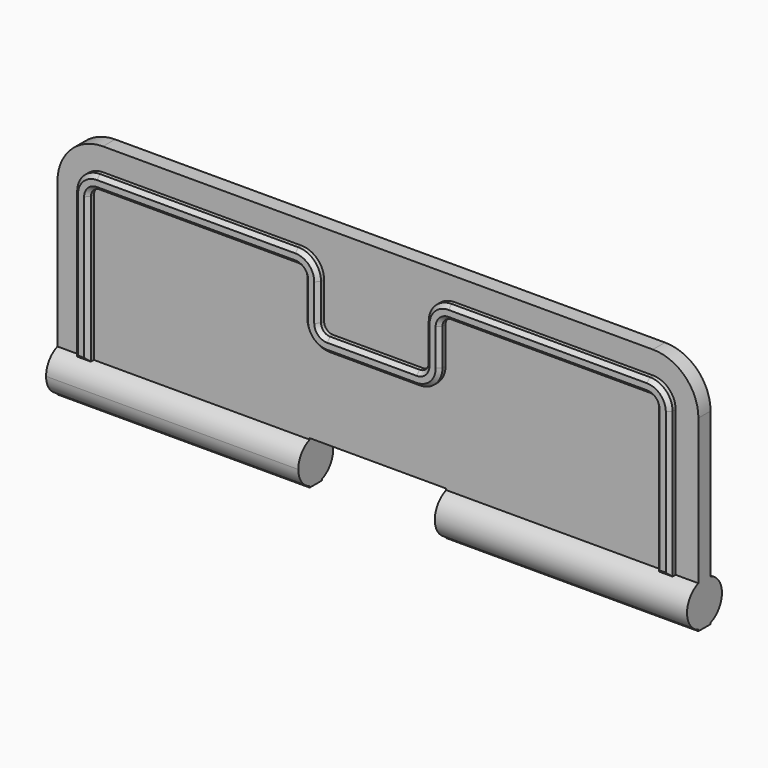
from build123d import *

# Parameters (mm, degrees)
F0_W     = 33.259
F0_H     = 5.75
F1_DEPTH = 2
F3_DEPTH = 33.259
F6_DEPTH = 33.259
F4_W     = 1.8128321722
F4_H     = 19.1795176684
F4_W_2   = 26.160747505
F4_H_2   = 1.8128321722
F4_H_3   = 4.8250346239
F4_W_3   = 5.911082495
F4_H_4   = 1.81283
F7_DEPTH = 1
F8_SIZE  = 0.5


# Not quite as in the source:
# - ends of sketch curves that miss each other by under 0.0002 mm in the source are joined
# - a pattern or mirror of a feature is missing from the dataset's text; its kind, count and spacing are read off the source's solid


with BuildPart() as f1:
    # F0 (on Front) → F1 (new body)
    with BuildSketch(Plane.XZ):
        with BuildLine():
            Line((36.259, 12.5), (-36.259, 12.5))
            ThreePointArc((-36.259, 12.5), (-40.5016406871, 10.7426406871), (-42.259, 6.5))
            Line((-42.259, 6.5), (-42.259, -12.5))
            Line((-42.259, -12.5), (-9, -12.5))
            Line((-9, -12.5), (-3.6677482234, -11.0712274426))
            Line((-3.6677482234, -11.0712274426), (3.6677482234, -11.0712274426))
            Line((3.6677482234, -11.0712274426), (9, -12.5))
            Line((9, -12.5), (42.259, -12.5))
            Line((42.259, -12.5), (42.259, 6.5))
            ThreePointArc((42.259, 6.5), (40.5016406871, 10.7426406871), (36.259, 12.5))
        make_face()
        with Locations((-25.6295, -15.375)):
            Rectangle(F0_W, F0_H)
        with Locations((25.6295, -15.375)):
            Rectangle(F0_W, F0_H)
        Polygon((-3.6677482234, -11.0712274426), (-9, -12.5), (9, -12.5), (3.6677482234, -11.0712274426), align=None)
    extrude(amount=F1_DEPTH)

    # F2 (on face) → F3 (join, through all)
    with BuildSketch(Plane(origin=(-42.259, 0, 0), x_dir=(0, -1, 0), z_dir=(-1, 0, 0))):
        with BuildLine():
            ThreePointArc((3.875, -15.375), (3.3601509486, -13.7332593079), (2, -12.6795176684))
            Line((2, -12.6795176684), (2, -18.0704823316))
            ThreePointArc((2, -18.0704823316), (3.3601509486, -17.0167406921), (3.875, -15.375))
        make_face()
        with BuildLine():
            Line((2, -18.0704823316), (2, -12.6795176684))
            ThreePointArc((2, -12.6795176684), (-1.875, -15.375), (2, -18.0704823316))
        make_face()
    extrude(amount=-F3_DEPTH)

    # F5 (on face) → F6 (join, through all)
    with BuildSketch(Plane.YZ.offset(42.259)):
        with BuildLine():
            ThreePointArc((0, -18.0704823316), (1.875, -15.375), (0, -12.6795176684))
            Line((0, -12.6795176684), (0, -12.5))
            Line((0, -12.5), (-2, -12.5))
            Line((-2, -12.5), (-2, -12.6795176684))
            ThreePointArc((-2, -12.6795176684), (-3.875, -15.375), (-2, -18.0704823316))
            Line((-2, -18.0704823316), (-2, -18.25))
            Line((-2, -18.25), (0, -18.25))
            Line((0, -18.25), (0, -18.0704823316))
        make_face()
    extrude(amount=-F6_DEPTH)

    # F4 (on face) → F7 (join)
    with BuildSketch(Plane.XZ.offset(2)):
        with Locations((-38.3525839139, -3.0897588342)):
            Rectangle(F4_W, F4_H)
        with BuildLine():
            ThreePointArc((-36.259, 9.5), (-38.3803203436, 8.6213203436), (-39.259, 6.5))
            Line((-39.259, 6.5), (-37.4461678278, 6.5))
            ThreePointArc((-37.4461678278, 6.5), (-37.0984544214, 7.3394544214), (-36.259, 7.6871678278))
            Line((-36.259, 7.6871678278), (-36.259, 9.5))
        make_face()
        with Locations((-23.1786262475, 8.5935839139)):
            Rectangle(F4_W_2, F4_H_2)
        with BuildLine():
            ThreePointArc((-7.098252495, 6.5), (-7.9769321514, 8.6213203436), (-10.098252495, 9.5))
            Line((-10.098252495, 9.5), (-10.098252495, 7.6871678278))
            ThreePointArc((-10.098252495, 7.6871678278), (-9.2587980736, 7.3394544214), (-8.9110846672, 6.5))
            Line((-8.9110846672, 6.5), (-7.098252495, 6.5))
        make_face()
        with Locations((-8.0046685811, 4.087482688)):
            Rectangle(F4_W, F4_H_3)
        with Locations((-2.9555412475, -0.4186196239)):
            Rectangle(F4_W_3, F4_H_4)
        with BuildLine():
            ThreePointArc((-5.911082495, 0.4877953761), (-6.7505384524, 0.8355094187), (-7.098252495, 1.6749653761))
            Line((-7.098252495, 1.6749653761), (-8.9110846672, 1.6749653761))
            ThreePointArc((-8.9110846672, 1.6749653761), (-8.0324028386, -0.4463549675), (-5.911082495, -1.3250346239))
            Line((-5.911082495, -1.3250346239), (-5.911082495, 0.4877953761))
        make_face()
    f7 = extrude(amount=F7_DEPTH)

    # F7_copies: F7 across plane
    add(f7.mirror(Plane(origin=(0, 0, 0), x_dir=(0, 0, 1), z_dir=(1, 0, 0))))

    # F8
    f8_edges = [f1.edges().sort_by_distance(p)[0] for p in [
        (39.259, -3, -3.089759),
        (38.352584, -3, -12.679518),
        (37.446168, -3, -3.089759),
        (37.098454, -3, 7.339454),
        (23.178626, -3, 7.687168),
        (9.258798, -3, 7.339454),
        (8.911085, -3, 4.087483),
        (8.032403, -3, -0.446355),
        (0, -3, -1.325035),
        (-8.032403, -3, -0.446355),
        (-8.911085, -3, 4.087483),
        (-9.258798, -3, 7.339454),
        (-23.178626, -3, 7.687168),
        (-37.098454, -3, 7.339454),
        (-37.446168, -3, -3.089759),
        (-38.352584, -3, -12.679518),
        (-39.259, -3, -3.089759),
        (-38.38032, -3, 8.62132),
        (-23.178626, -3, 9.5),
        (-7.976932, -3, 8.62132),
        (-7.098252, -3, 4.087483),
        (-6.750538, -3, 0.835509),
        (0, -3, 0.487795),
        (6.750538, -3, 0.835509),
        (7.098252, -3, 4.087483),
        (7.976932, -3, 8.62132),
        (23.178626, -3, 9.5),
        (38.38032, -3, 8.62132),
    ]]
    chamfer(f8_edges, length=F8_SIZE)


solid = f1.part
